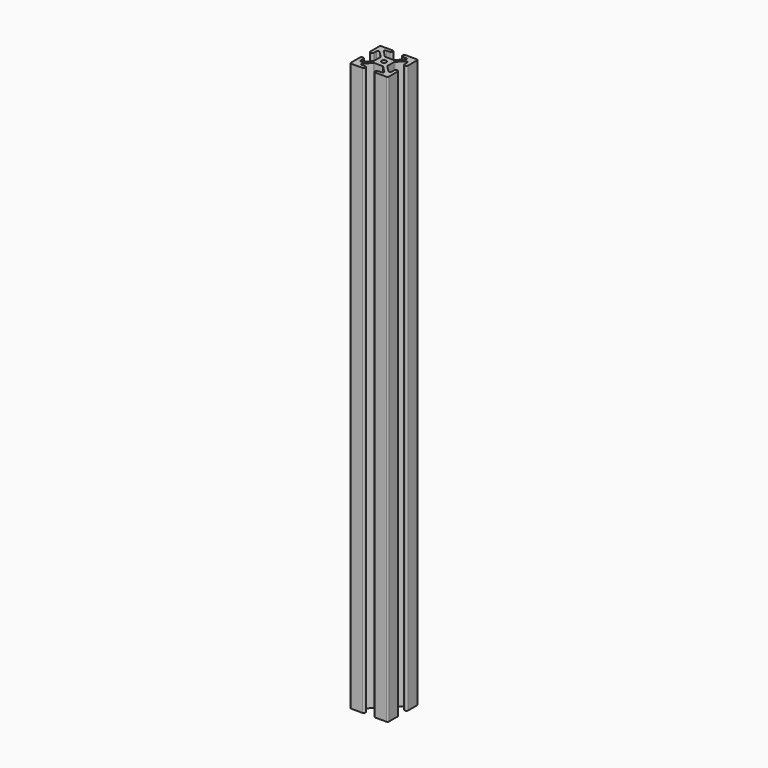
from build123d import *

# Parameters (mm, degrees)
F1_R     = 1.6335205603
F2_DEPTH = 381


# Not quite as in the source:
# - a variable given as a bare number and used for a length is read in inches; the dataset says mm whatever the document's units were


with BuildPart() as f2:
    # F1 (on Top) → F2 (new body)
    with BuildSketch(Plane.XY):
        with BuildLine():
            Line((-2.590399578, -4.5212), (2.590399578, -4.5212))
            ThreePointArc((2.590399578, -4.5212), (2.9306051494, -4.5888710956), (3.2190175065, -4.7815820715))
            Line((3.2190175065, -4.7815820715), (7.2830175065, -8.8455820715))
            ThreePointArc((7.2830175065, -8.8455820715), (7.4757284824, -9.8144055714), (6.654399578, -10.3632))
            Line((6.654399578, -10.3632), (4.4209109178, -10.3632))
            ThreePointArc((4.4209109178, -10.3632), (3.5947273547, -10.7054164369), (3.2525109178, -11.5316))
            ThreePointArc((3.2525109178, -11.5316), (3.5947273547, -12.3577835631), (4.4209109178, -12.7))
            Line((4.4209109178, -12.7), (11.811, -12.7))
            ThreePointArc((11.811, -12.7), (12.4396179285, -12.4396179285), (12.7, -11.811))
            Line((12.7, -11.811), (12.7, -4.4209109178))
            ThreePointArc((12.7, -4.4209109178), (12.3577835631, -3.5947273547), (11.5316, -3.2525109178))
            ThreePointArc((11.5316, -3.2525109178), (10.7054164369, -3.5947273547), (10.3632, -4.4209109178))
            Line((10.3632, -4.4209109178), (10.3632, -6.654399578))
            ThreePointArc((10.3632, -6.654399578), (9.8144055714, -7.4757284824), (8.8455820715, -7.2830175065))
            Line((8.8455820715, -7.2830175065), (4.7815820715, -3.2190175065))
            ThreePointArc((4.7815820715, -3.2190175065), (4.5888710956, -2.9306051494), (4.5212, -2.590399578))
            Line((4.5212, -2.590399578), (4.5212, 2.590399578))
            ThreePointArc((4.5212, 2.590399578), (4.5888710956, 2.9306051494), (4.7815820715, 3.2190175065))
            Line((4.7815820715, 3.2190175065), (8.8455820715, 7.2830175065))
            ThreePointArc((8.8455820715, 7.2830175065), (9.8144055714, 7.4757284824), (10.3632, 6.654399578))
            Line((10.3632, 6.654399578), (10.3632, 4.4209109178))
            ThreePointArc((10.3632, 4.4209109178), (10.7054164369, 3.5947273547), (11.5316, 3.2525109178))
            ThreePointArc((11.5316, 3.2525109178), (12.3577835631, 3.5947273547), (12.7, 4.4209109178))
            Line((12.7, 4.4209109178), (12.7, 11.811))
            ThreePointArc((12.7, 11.811), (12.4396179285, 12.4396179285), (11.811, 12.7))
            Line((11.811, 12.7), (4.4209109178, 12.7))
            ThreePointArc((4.4209109178, 12.7), (3.5947273547, 12.3577835631), (3.2525109178, 11.5316))
            ThreePointArc((3.2525109178, 11.5316), (3.5947273547, 10.7054164369), (4.4209109178, 10.3632))
            Line((4.4209109178, 10.3632), (6.654399578, 10.3632))
            ThreePointArc((6.654399578, 10.3632), (7.4757284824, 9.8144055714), (7.2830175065, 8.8455820715))
            Line((7.2830175065, 8.8455820715), (3.2190175065, 4.7815820715))
            ThreePointArc((3.2190175065, 4.7815820715), (2.9306051494, 4.5888710956), (2.590399578, 4.5212))
            Line((2.590399578, 4.5212), (-2.590399578, 4.5212))
            ThreePointArc((-2.590399578, 4.5212), (-2.9306051494, 4.5888710956), (-3.2190175065, 4.7815820715))
            Line((-3.2190175065, 4.7815820715), (-7.2830175065, 8.8455820715))
            ThreePointArc((-7.2830175065, 8.8455820715), (-7.4757284824, 9.8144055714), (-6.654399578, 10.3632))
            Line((-6.654399578, 10.3632), (-4.4209109178, 10.3632))
            ThreePointArc((-4.4209109178, 10.3632), (-3.5947273547, 10.7054164369), (-3.2525109178, 11.5316))
            ThreePointArc((-3.2525109178, 11.5316), (-3.5947273547, 12.3577835631), (-4.4209109178, 12.7))
            Line((-4.4209109178, 12.7), (-11.811, 12.7))
            ThreePointArc((-11.811, 12.7), (-12.4396179285, 12.4396179285), (-12.7, 11.811))
            Line((-12.7, 11.811), (-12.7, 4.4209109178))
            ThreePointArc((-12.7, 4.4209109178), (-12.3379947006, 3.575401517), (-11.4762989613, 3.2538203664))
            ThreePointArc((-11.4762989613, 3.2538203664), (-10.6860905992, 3.6145162172), (-10.3632, 4.4209109178))
            Line((-10.3632, 4.4209109178), (-10.3632, 6.654399578))
            ThreePointArc((-10.3632, 6.654399578), (-9.8144055714, 7.4757284824), (-8.8455820715, 7.2830175065))
            Line((-8.8455820715, 7.2830175065), (-4.7815820715, 3.2190175065))
            ThreePointArc((-4.7815820715, 3.2190175065), (-4.5888710956, 2.9306051494), (-4.5212, 2.590399578))
            Line((-4.5212, 2.590399578), (-4.5212, -2.590399578))
            ThreePointArc((-4.5212, -2.590399578), (-4.5888710956, -2.9306051494), (-4.7815820715, -3.2190175065))
            Line((-4.7815820715, -3.2190175065), (-8.8455820715, -7.2830175065))
            ThreePointArc((-8.8455820715, -7.2830175065), (-9.8144055714, -7.4757284824), (-10.3632, -6.654399578))
            Line((-10.3632, -6.654399578), (-10.3632, -4.4209109178))
            ThreePointArc((-10.3632, -4.4209109178), (-10.7252052994, -3.575401517), (-11.5869010387, -3.2538203664))
            ThreePointArc((-11.5869010387, -3.2538203664), (-12.3771094008, -3.6145162172), (-12.7, -4.4209109178))
            Line((-12.7, -4.4209109178), (-12.7, -11.811))
            ThreePointArc((-12.7, -11.811), (-12.4396179285, -12.4396179285), (-11.811, -12.7))
            Line((-11.811, -12.7), (-4.4209109178, -12.7))
            ThreePointArc((-4.4209109178, -12.7), (-3.5947273547, -12.3577835631), (-3.2525109178, -11.5316))
            ThreePointArc((-3.2525109178, -11.5316), (-3.5947273547, -10.7054164369), (-4.4209109178, -10.3632))
            Line((-4.4209109178, -10.3632), (-6.654399578, -10.3632))
            ThreePointArc((-6.654399578, -10.3632), (-7.4757284824, -9.8144055714), (-7.2830175065, -8.8455820715))
            Line((-7.2830175065, -8.8455820715), (-3.2190175065, -4.7815820715))
            ThreePointArc((-3.2190175065, -4.7815820715), (-2.9306051494, -4.5888710956), (-2.590399578, -4.5212))
        make_face()
        Circle(F1_R, mode=Mode.SUBTRACT)
    extrude(amount=F2_DEPTH)


solid = f2.part
